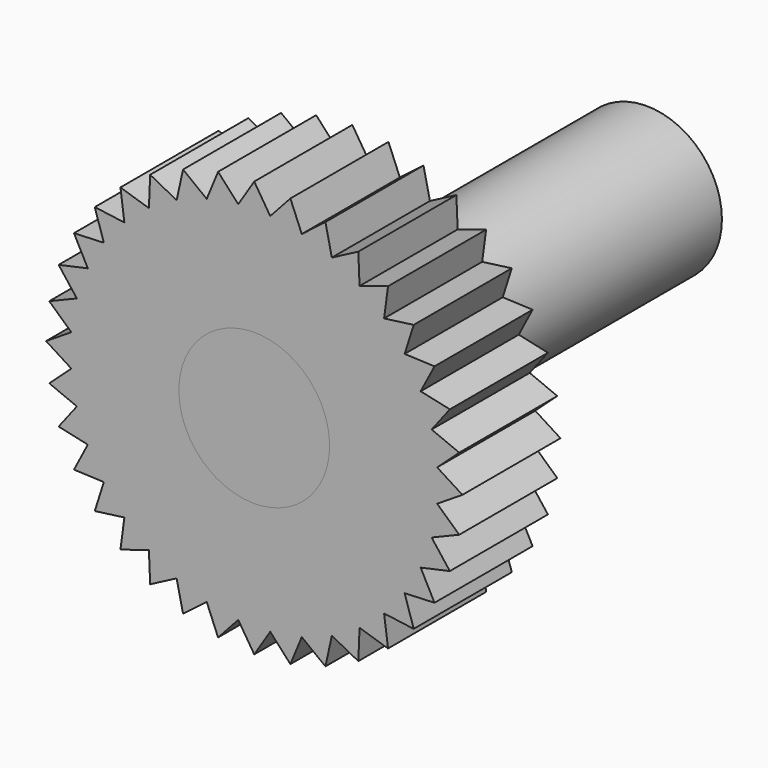
from build123d import *

# Parameters (mm, degrees)
F0_R            = 15.6138441185
F1_DEPTH        = 101.6
F2_R            = 38.0450416099
F2_R_2          = 15.6138441185
F3_DEPTH        = 25.4
F5_DEPTH        = 25.4
F5_COPIES_COUNT = 36


# Not quite as in the source:
# - a pattern or mirror of a feature is missing from the dataset's text; its kind, count and spacing are read off the source's solid


with BuildPart() as f1:
    # F0 (on Front) → F1 (new body)
    with BuildSketch(Plane.XZ):
        Circle(F0_R)
    extrude(amount=F1_DEPTH)


with BuildPart() as f3:
    # F2 (on face) → F3 (new body)
    with BuildSketch(Plane.XZ.offset(101.6)):
        Circle(F2_R)
        Circle(F2_R_2, mode=Mode.SUBTRACT)
    extrude(amount=-F3_DEPTH)

    # F4 (on face) → F5 (join, through all)
    with BuildSketch(Plane.XZ.offset(101.6)):
        with BuildLine():
            Line((0, 43.1250416099), (-3.3158438594, 37.9002687404))
            ThreePointArc((-3.3158438594, 37.9002687404), (0, 38.0450416099), (3.3158438594, 37.9002687404))
            Line((3.3158438594, 37.9002687404), (0, 43.1250416099))
        make_face()
    f5 = extrude(amount=-F5_DEPTH)

    # F5_copies: F5 ×36 about axis
    f5_copies_axis = Axis((0, 0, 0), (0, 1, 0))
    for i in range(1, F5_COPIES_COUNT):
        add(f5.rotate(f5_copies_axis, i * 360 / F5_COPIES_COUNT))


solid = Compound([f1.part, f3.part])
